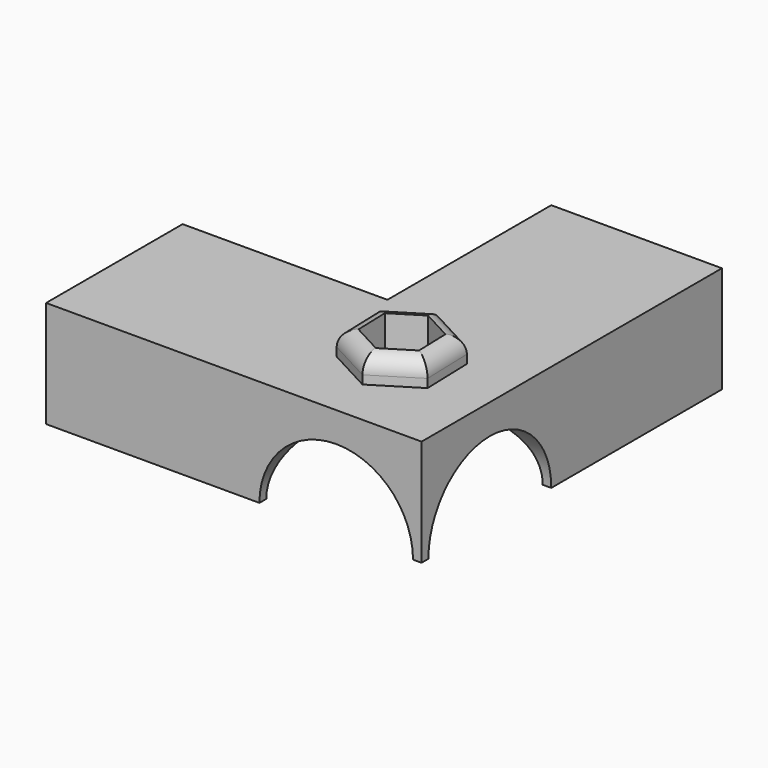
from build123d import *

# Parameters (mm, degrees)
F1_DEPTH      = 25
F2_R          = 9
F3_DEPTH      = 44.001
F4_R          = 9
F5_DEPTH      = 44.001
F7_DEPTH      = 44.0010001
F8_R          = 2.5
F9_DEPTH      = 2
F10_DEPTH     = 3
F11_T1_DEPTH  = 16
F11_T3_DEPTH  = 16
F11_T5_DEPTH  = 16
F11_T7_DEPTH  = 16
F11_T9_DEPTH  = 16
F11_T11_DEPTH = 16


# Not quite as in the source:
# - a fillet or chamfer that OpenCascade refuses, or shapes differently, is made with other operations: its cross-section is extruded or revolved along the edge and cut away or added


with BuildPart() as f1:
    # F0 (on Top) → F1 (new body)
    with BuildSketch(Plane.XY):
        with BuildLine():
            Line((6.9382145885, -6.9382145885), (0, 0))
            Line((0, 0), (-24, 0))
            Line((-24, 0), (-24, -20))
            Line((-24, -20), (20, -20))
            Line((20, -20), (10.4737484944, -10.4737484944))
            ThreePointArc((10.4737484944, -10.4737484944), (6.9382145885, -10.4737484944), (6.9382145885, -6.9382145885))
        make_face()
        with BuildLine():
            Line((20, 24), (0, 24))
            Line((0, 24), (0, 0))
            Line((0, 0), (6.9382145885, -6.9382145885))
            ThreePointArc((6.9382145885, -6.9382145885), (9.6626901223, -6.3962827101), (11.2059815414, -8.7059815414))
            ThreePointArc((11.2059815414, -8.7059815414), (11.0156803727, -9.6626901223), (10.4737484944, -10.4737484944))
            Line((10.4737484944, -10.4737484944), (20, -20))
            Line((20, -20), (20, 24))
        make_face()
    extrude(amount=F1_DEPTH)

    # F2 (on face) → F3 (cut, through all)
    with BuildSketch(Plane(origin=(-24, 0, 0), x_dir=(0, -1, 0), z_dir=(-1, 0, 0))):
        with Locations((10, 12.5)):
            Circle(F2_R)
    extrude(amount=-F3_DEPTH, mode=Mode.SUBTRACT)

    # F4 (on face) → F5 (cut, through all)
    with BuildSketch(Plane(origin=(0, 24, 0), x_dir=(-1, 0, 0), z_dir=(0, 1, 0))):
        with Locations((-10, 12.5)):
            Circle(F4_R)
    extrude(amount=-F5_DEPTH, mode=Mode.SUBTRACT)

    # F6 (on face) → F7 (cut, through all)
    with BuildSketch(Plane.XZ.offset(20)):
        with BuildLine():
            Line((20, 12.5), (19, 12.5))
            ThreePointArc((19, 12.5), (10, 3.5), (1, 12.5))
            Line((1, 12.5), (-24, 12.5))
            Line((-24, 12.5), (-24, 0))
            Line((-24, 0), (20, 0))
            Line((20, 0), (20, 12.5))
        make_face()
    extrude(amount=-F7_DEPTH, mode=Mode.SUBTRACT)

    # F8 (on face) → F9 (cut)
    with BuildSketch(Plane.XY.offset(25)):
        Polygon((5.0551444558, -6.7069682099), (5.1807740761, -10.704994873), (8.7059815414, -12.5952097618), (12.1055593865, -10.4873979877), (11.9799297662, -6.4893713246), (8.4547223009, -4.5991564357), align=None)
        with Locations((8.7059815414, -8.7059815414)):
            Circle(F8_R, mode=Mode.SUBTRACT)
    extrude(amount=-F9_DEPTH, mode=Mode.SUBTRACT)

    # F8 (on face) → F10 (join)
    with BuildSketch(Plane.XY.offset(25)):
        Polygon((3.229725913, -5.7074615441), (3.4181703434, -11.7045015387), (8.7059815414, -14.5398238721), (13.805348309, -11.3781062108), (13.6169038786, -5.3810662162), (8.3290926806, -2.5457438829), align=None)
        Polygon((8.7059815414, -12.5952097618), (5.1807740761, -10.704994873), (5.0551444558, -6.7069682099), (8.4547223009, -4.5991564357), (11.9799297662, -6.4893713246), (12.1055593865, -10.4873979877), align=None, mode=Mode.SUBTRACT)
    extrude(amount=F10_DEPTH)

    # F11: fillet of radius 2 on 6 edges, made by hand

    # F11_s2 → F11_t1 (cut)
    with BuildSketch(Plane(origin=(17.2236751454, -9.2353279974, 0), x_dir=(0, 0, 1), z_dir=(-0.8813018663, 0.4725537222, 0))):
        with BuildLine():
            ThreePointArc((26, 1.6923749137), (27.4142135624, 1.1065884761), (28, -0.3076250863))
            Line((28, -0.3076250863), (28, 1.6923749137))
            Line((28, 1.6923749137), (26, 1.6923749137))
        make_face()
    extrude(amount=F11_T1_DEPTH, mode=Mode.SUBTRACT)

    # F11_s4 → F11_t3 (cut)
    with BuildSketch(Plane(origin=(0.5278354617, -16.7977921518, 0), x_dir=(0, 0, 1), z_dir=(-0.0314074051, 0.9995066658, 0))):
        with BuildLine():
            ThreePointArc((28, 11.4411808674), (27.4142135624, 12.8553944297), (26, 13.4411808674))
            Line((26, 13.4411808674), (28, 13.4411808674))
            Line((28, 13.4411808674), (28, 11.4411808674))
        make_face()
    extrude(amount=F11_T3_DEPTH, mode=Mode.SUBTRACT)

    # F11_s6 → F11_t5 (cut)
    with BuildSketch(Plane(origin=(-4.4726864595, -2.7731623193, 0), x_dir=(0, 0, 1), z_dir=(0.8498944613, 0.5269529435, 0))):
        with BuildLine():
            ThreePointArc((28, 14.9449583763), (27.4142135624, 16.3591719387), (26, 16.9449583763))
            Line((26, 16.9449583763), (28, 16.9449583763))
            Line((28, 16.9449583763), (28, 14.9449583763))
        make_face()
    extrude(amount=F11_T5_DEPTH, mode=Mode.SUBTRACT)

    # F11_s8 → F11_t7 (cut)
    with BuildSketch(Plane(origin=(3.122845284, -1.6744684418, 0), x_dir=(0, 0, 1), z_dir=(0.8813018663, -0.4725537222, 0))):
        with BuildLine():
            ThreePointArc((28, 6.6999299317), (27.4142135624, 8.1141434941), (26, 8.6999299317))
            Line((26, 8.6999299317), (28, 8.6999299317))
            Line((28, 8.6999299317), (28, 6.6999299317))
        make_face()
    extrude(amount=F11_T7_DEPTH, mode=Mode.SUBTRACT)

    # F11_s10 → F11_t9 (cut)
    with BuildSketch(Plane(origin=(0.0253169806, -0.8056854995, 0), x_dir=(0, 0, 1), z_dir=(0.0314074051, -0.9995066658, 0))):
        with BuildLine():
            ThreePointArc((28, -5.048876022), (27.4142135624, -3.6346624596), (26, -3.048876022))
            Line((26, -3.048876022), (28, -3.048876022))
            Line((28, -3.048876022), (28, -5.048876022))
        make_face()
    extrude(amount=F11_T9_DEPTH, mode=Mode.SUBTRACT)

    # F11_s12 → F11_t11 (cut)
    with BuildSketch(Plane(origin=(9.1256249208, 5.6580847774, 0), x_dir=(0, 0, 1), z_dir=(-0.8498944613, -0.5269529435, 0))):
        with BuildLine():
            ThreePointArc((28, -8.5526535309), (27.4142135624, -7.1384399686), (26, -6.5526535309))
            Line((26, -6.5526535309), (28, -6.5526535309))
            Line((28, -6.5526535309), (28, -8.5526535309))
        make_face()
    extrude(amount=F11_T11_DEPTH, mode=Mode.SUBTRACT)


solid = f1.part
